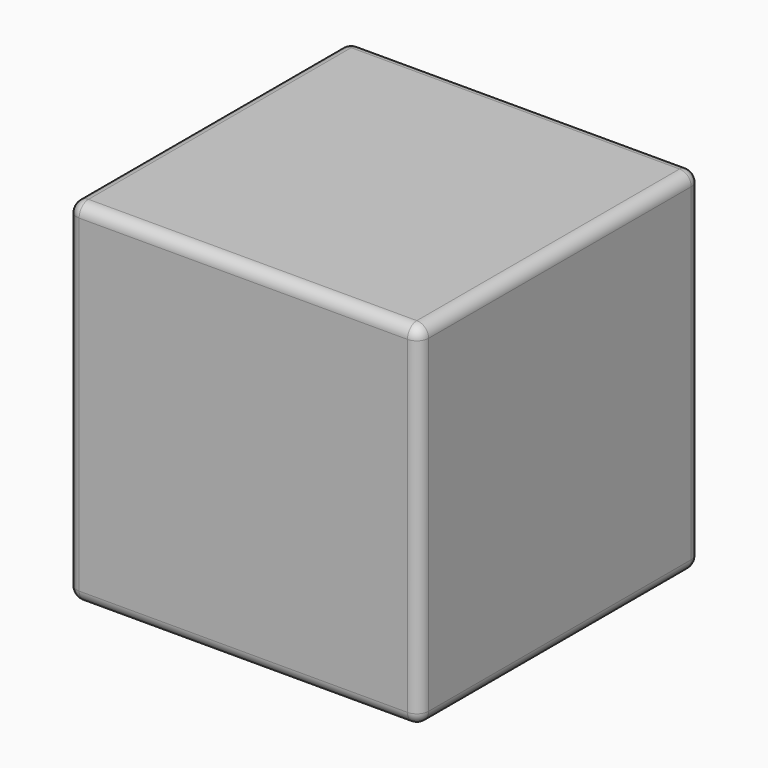
from build123d import *

# Parameters (mm, degrees)
F0_W     = 15
F0_H     = 15
F1_DEPTH = 15
F2_R     = 1.5
F3_DEPTH = 0.5
F4_R     = 0.5
F5_R     = 0.24999


# Not quite as in the source:
# - a fillet or chamfer is up to 0.001 mm smaller than in the source, because OpenCascade refuses the exact size
# - a feature names something its author has since deleted; it is built from what else it names


with BuildPart() as f1:
    # F0 (on Top) → F1 (new body)
    with BuildSketch(Plane.XY):
        with Locations((-2.0319856703, -2.0552466768)):
            Rectangle(F0_W, F0_H)
    extrude(amount=F1_DEPTH)

    # F2 (on face) → F3 (cut)
    with BuildSketch(Plane(origin=(0, 0, 0), x_dir=(1, 0, 0), z_dir=(0, 0, -1))):
        with Locations((-2.0319856703, 2.0552456845)):
            Circle(F2_R)
    extrude(amount=-F3_DEPTH, mode=Mode.SUBTRACT)

    # F4
    f4_edges = [f1.edges().sort_by_distance(p)[0] for p in [
        (5.468014, 5.444753, 7.5),
        (-2.031986, 5.444753, 0),
        (-2.031986, 5.444753, 15),
        (-9.531986, 5.444753, 7.5),
        (5.468014, -2.055247, 0),
        (5.468014, -2.055247, 15),
        (5.468014, -9.555247, 7.5),
        (-9.531986, -2.055247, 0),
        (-2.031986, -9.555247, 0),
        (-9.531986, -2.055247, 15),
        (-9.531986, -9.555247, 7.5),
        (-2.031986, -9.555247, 15),
    ]]
    fillet(f4_edges, radius=F4_R)

    # F5 (radius 0.25 in the source; OpenCascade refuses exactly that, so slightly less here)
    f5_edges = [f1.edges().sort_by_distance(p)[0] for p in [
        (-3.531986, -2.055246, 0.5),
        (-3.531986, -2.055246, 0),
    ]]
    fillet(f5_edges, radius=F5_R)


solid = f1.part
